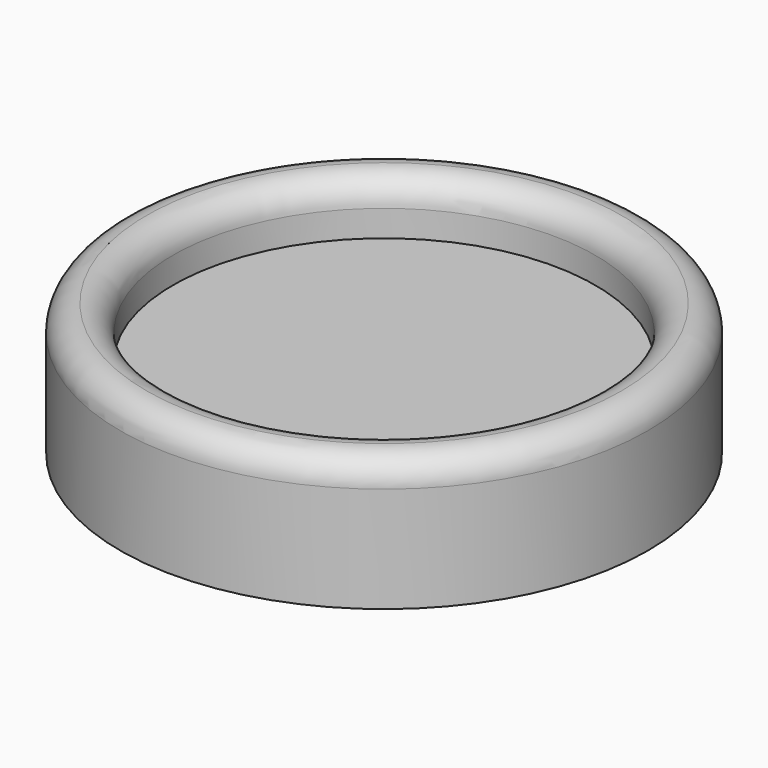
from build123d import *

# Parameters (mm, degrees)
F0_R     = 10
F1_DEPTH = 5
F2_R     = 8
F3_DEPTH = 2
F4_R     = 0.99999


# Not quite as in the source:
# - a fillet or chamfer is up to 0.001 mm smaller than in the source, because OpenCascade refuses the exact size


with BuildPart() as f1:
    # F0 (on Top) → F1 (new body)
    with BuildSketch(Plane.XY):
        Circle(F0_R)
    extrude(amount=F1_DEPTH)

    # F2 (on face) → F3 (cut)
    with BuildSketch(Plane.XY.offset(5)):
        Circle(F2_R)
    extrude(amount=-F3_DEPTH, mode=Mode.SUBTRACT)

    # F4 (radius 1 in the source; OpenCascade refuses exactly that, so slightly less here)
    f4_edges = [f1.edges().sort_by_distance(p)[0] for p in [
        (-10, 0, 5),
        (-8, 0, 5),
    ]]
    fillet(f4_edges, radius=F4_R)


solid = f1.part
